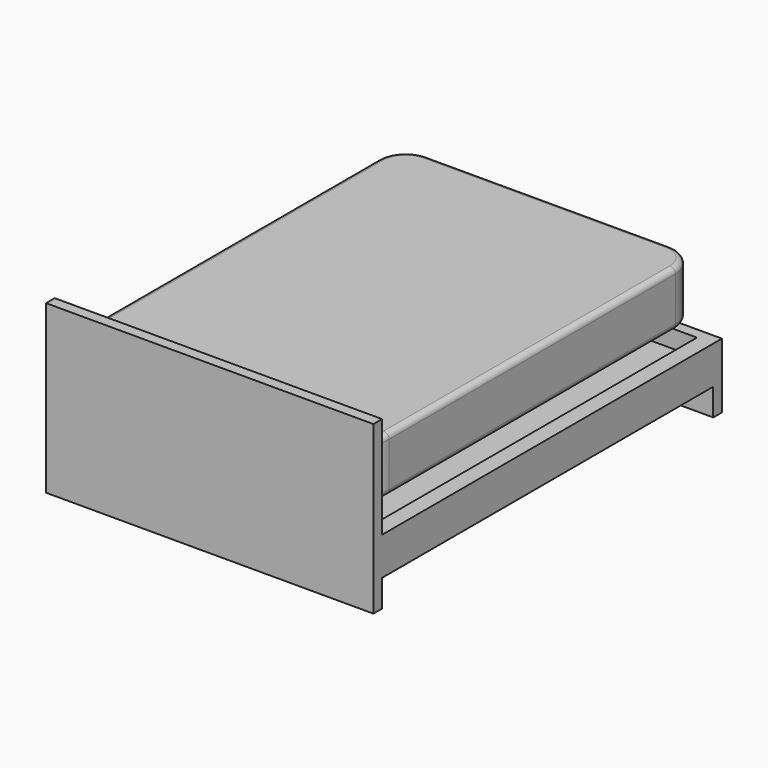
from build123d import *

# Parameters (mm, degrees)
F0_W         = 1371.6
F0_H         = 1905
F1_DEPTH     = 254
F2_R         = 25.4
F3_T1_DEPTH  = 254
F3_T4_ANGLE  = 90
F3_T6_ANGLE  = 90
F3_T8_ANGLE  = 90
F3_T10_ANGLE = 90
F3_T12_ANGLE = 90
F3_T14_ANGLE = 90
F3_T16_ANGLE = 90
F3_T18_ANGLE = 90
F4_W         = 1510
F4_H         = 770
F4_W_2       = 1117.6
F4_H_2       = 203.2
F5_DEPTH     = 50
F6_W         = 75
F6_H         = 175
F7_DEPTH     = 1910
F8_W         = 75
F8_H         = 175
F9_DEPTH     = 50
F11_START    = -80
F11_DEPTH    = 20


# Not quite as in the source:
# - a fillet or chamfer that OpenCascade refuses, or shapes differently, is made with other operations: its cross-section is extruded or revolved along the edge and cut away or added


with BuildPart() as f1:
    # F0 (on Top) → F1 (new body)
    with BuildSketch(Plane.XY):
        Rectangle(F0_W, F0_H)
    extrude(amount=F1_DEPTH)

    # F2
    f2_edges = [f1.edges().sort_by_distance(p)[0] for p in [
        (-685.8, 0, 254),
        (0, 952.5, 254),
        (685.8, 0, 254),
        (0, -952.5, 254),
        (685.8, 0, 0),
        (0, 952.5, 0),
        (-685.8, 0, 0),
        (0, -952.5, 0),
    ]]
    fillet(f2_edges, radius=F2_R)

    # F3: fillet of radius 127 on 4 edges, made by hand

    # F3_s2 → F3_t1 (cut)
    with BuildSketch(Plane.XY):
        with BuildLine():
            ThreePointArc((685.8, -825.5), (648.6025612107, -915.3025612107), (558.8, -952.5))
            Line((558.8, -952.5), (685.8, -952.5))
            Line((685.8, -952.5), (685.8, -825.5))
        make_face()
        with BuildLine():
            ThreePointArc((685.8, 825.5), (648.6025612107, 915.3025612107), (558.8, 952.5))
            Line((558.8, 952.5), (685.8, 952.5))
            Line((685.8, 952.5), (685.8, 825.5))
        make_face()
        with BuildLine():
            ThreePointArc((-558.8, 952.5), (-648.6025612107, 915.3025612107), (-685.8, 825.5))
            Line((-685.8, 825.5), (-685.8, 952.5))
            Line((-685.8, 952.5), (-558.8, 952.5))
        make_face()
        with BuildLine():
            ThreePointArc((-558.8, -952.5), (-648.6025612107, -915.3025612107), (-685.8, -825.5))
            Line((-685.8, -825.5), (-685.8, -952.5))
            Line((-685.8, -952.5), (-558.8, -952.5))
        make_face()
    extrude(amount=F3_T1_DEPTH, mode=Mode.SUBTRACT)

    # F3_s3 → F3_t4 (revolve, cut)
    with BuildSketch(Plane.YZ.offset(-558.8)):
        with BuildLine():
            ThreePointArc((-927.1, 0), (-945.0605122421, 7.4394877579), (-952.5, 25.4))
            Line((-952.5, 25.4), (-952.5, 0))
            Line((-952.5, 0), (-927.1, 0))
        make_face()
    revolve(axis=Axis((-558.8, -825.5, 0), (0, 0, -1)), revolution_arc=F3_T4_ANGLE, mode=Mode.SUBTRACT)

    # F3_s5 → F3_t6 (revolve, cut)
    with BuildSketch(Plane.XZ.offset(825.5)):
        with BuildLine():
            ThreePointArc((-660.4, 254), (-678.3605122421, 246.5605122421), (-685.8, 228.6))
            Line((-685.8, 228.6), (-685.8, 254))
            Line((-685.8, 254), (-660.4, 254))
        make_face()
    revolve(axis=Axis((-558.8, -825.5, 254), (0, 0, 1)), revolution_arc=F3_T6_ANGLE, mode=Mode.SUBTRACT)

    # F3_s7 → F3_t8 (revolve, cut)
    with BuildSketch(Plane.XZ.offset(-825.5)):
        with BuildLine():
            ThreePointArc((-660.4, 0), (-678.3605122421, 7.4394877579), (-685.8, 25.4))
            Line((-685.8, 25.4), (-685.8, 0))
            Line((-685.8, 0), (-660.4, 0))
        make_face()
    revolve(axis=Axis((-558.8, 825.5, 0), (0, 0, -1)), revolution_arc=F3_T8_ANGLE, mode=Mode.SUBTRACT)

    # F3_s9 → F3_t10 (revolve, cut)
    with BuildSketch(Plane.YZ.offset(-558.8)):
        with BuildLine():
            ThreePointArc((927.1, 254), (945.0605122421, 246.5605122421), (952.5, 228.6))
            Line((952.5, 228.6), (952.5, 254))
            Line((952.5, 254), (927.1, 254))
        make_face()
    revolve(axis=Axis((-558.8, 825.5, 254), (0, 0, 1)), revolution_arc=F3_T10_ANGLE, mode=Mode.SUBTRACT)

    # F3_s11 → F3_t12 (revolve, cut)
    with BuildSketch(Plane.YZ.offset(558.8)):
        with BuildLine():
            ThreePointArc((927.1, 0), (945.0605122421, 7.4394877579), (952.5, 25.4))
            Line((952.5, 25.4), (952.5, 0))
            Line((952.5, 0), (927.1, 0))
        make_face()
    revolve(axis=Axis((558.8, 825.5, 0), (0, 0, -1)), revolution_arc=F3_T12_ANGLE, mode=Mode.SUBTRACT)

    # F3_s13 → F3_t14 (revolve, cut)
    with BuildSketch(Plane.XZ.offset(-825.5)):
        with BuildLine():
            ThreePointArc((660.4, 254), (678.3605122421, 246.5605122421), (685.8, 228.6))
            Line((685.8, 228.6), (685.8, 254))
            Line((685.8, 254), (660.4, 254))
        make_face()
    revolve(axis=Axis((558.8, 825.5, 254), (0, 0, 1)), revolution_arc=F3_T14_ANGLE, mode=Mode.SUBTRACT)

    # F3_s15 → F3_t16 (revolve, cut)
    with BuildSketch(Plane.XZ.offset(825.5)):
        with BuildLine():
            ThreePointArc((660.4, 0), (678.3605122421, 7.4394877579), (685.8, 25.4))
            Line((685.8, 25.4), (685.8, 0))
            Line((685.8, 0), (660.4, 0))
        make_face()
    revolve(axis=Axis((558.8, -825.5, 0), (0, 0, -1)), revolution_arc=F3_T16_ANGLE, mode=Mode.SUBTRACT)

    # F3_s17 → F3_t18 (revolve, cut)
    with BuildSketch(Plane.YZ.offset(558.8)):
        with BuildLine():
            ThreePointArc((-927.1, 254), (-945.0605122421, 246.5605122421), (-952.5, 228.6))
            Line((-952.5, 228.6), (-952.5, 254))
            Line((-952.5, 254), (-927.1, 254))
        make_face()
    revolve(axis=Axis((558.8, -825.5, 254), (0, 0, 1)), revolution_arc=F3_T18_ANGLE, mode=Mode.SUBTRACT)


with BuildPart() as f5:
    # F4 (on face) → F5 (new body)
    with BuildSketch(Plane.XZ.offset(952.5)):
        Rectangle(F4_W, F4_H)
        with Locations((0, 127)):
            Rectangle(F4_W_2, F4_H_2, mode=Mode.SUBTRACT)
        with Locations((0, 127)):
            Rectangle(F4_W_2, F4_H_2)
    extrude(amount=F5_DEPTH)

    # F6 (on face) → F7 (join)
    with BuildSketch(Plane(origin=(0, -952.5, 0), x_dir=(-1, 0, 0), z_dir=(0, 1, 0))):
        with Locations((-717.5, -172.5)):
            Rectangle(F6_W, F6_H)
        with Locations((717.5, -172.5)):
            Rectangle(F6_W, F6_H)
    extrude(amount=F7_DEPTH)

    # F8 (on face) → F9 (join)
    with BuildSketch(Plane(origin=(0, 957.5, 0), x_dir=(-1, 0, 0), z_dir=(0, 1, 0))):
        with Locations((-717.5, -172.5)):
            Rectangle(F8_W, F8_H)
        Polygon((755, -85), (-680, -85), (-680, -260), (-755, -260), (-755, -385), (755, -385), align=None)
    extrude(amount=F9_DEPTH)

    # F10 (on face) → F11 (join)
    with BuildSketch(Plane.XY.offset(-85).offset(F11_START)):
        Polygon((680, 955), (-680, 955), (-680, -952.5), (-680, -955), (680, -955), (680, -952.5), align=None)
    extrude(amount=-F11_DEPTH)


solid = Compound([f1.part, f5.part])
